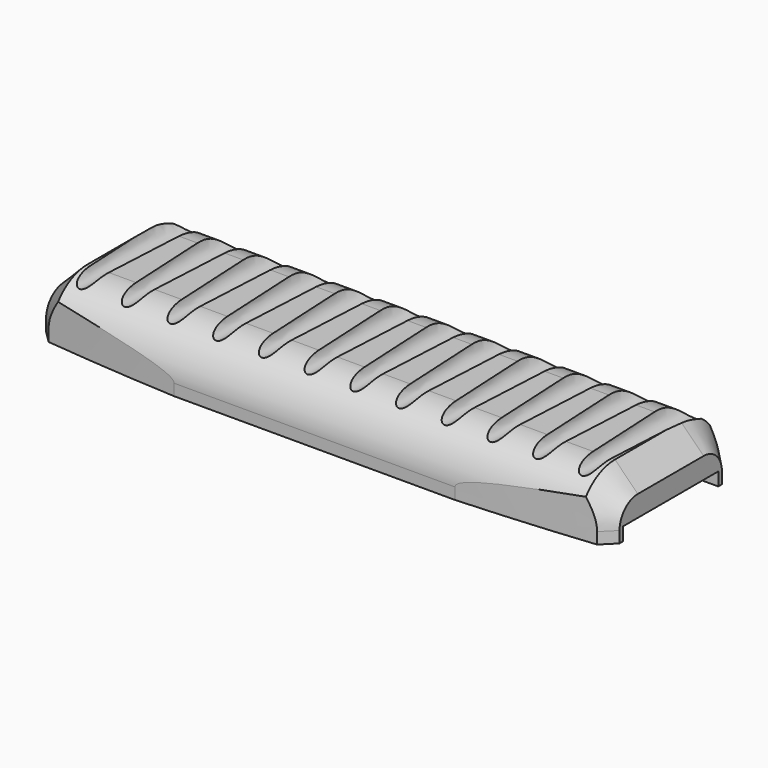
from build123d import *

# Parameters (mm, degrees)
F0_W         = 125.463343301
F0_H         = 38
F1_DEPTH     = 12.5
F2_W         = 26
F2_H         = 2.9014106728
F3_DEPTH     = 98.4
F4_R         = 10
F5_R         = 1.5
F6_DEPTH     = 42.5
F6_TAPER     = -3
F7_T1_DEPTH  = 15.3584149398
F7_T3_DEPTH  = 18
F7_T6_ANGLE  = 90
F7_T8_ANGLE  = 90
F7_T10_ANGLE = 90
F7_T12_ANGLE = 90
F9_DEPTH     = 25


# Not quite as in the source:
# - a fillet or chamfer that OpenCascade refuses, or shapes differently, is made with other operations: its cross-section is extruded or revolved along the edge and cut away or added


with BuildPart() as f1:
    # F0 (on Top) → F1 (new body)
    with BuildSketch(Plane.XY):
        with Locations((20.3044549349, 19)):
            Rectangle(F0_W, F0_H)
    extrude(amount=F1_DEPTH)

    # F2 (on Right) → F3 (cut, symmetric)
    with BuildSketch(Plane.YZ):
        with Locations((19, 1.4507053364)):
            Rectangle(F2_W, F2_H)
    extrude(amount=F3_DEPTH, both=True, mode=Mode.SUBTRACT)

    # F4
    f4_edges = [f1.edges().sort_by_distance(p)[0] for p in [
        (20.304455, 38, 12.5),
        (20.304455, 0, 12.5),
    ]]
    fillet(f4_edges, radius=F4_R)

    # F5 (on Front) → F6 (cut)
    with BuildSketch(Plane.XZ):
        with Locations((-34.7272167156, 12.6250582502)):
            Circle(F5_R)
        with Locations((-24.7272167156, 12.5)):
            Circle(F5_R)
        with Locations((-14.7272167156, 12.5)):
            Circle(F5_R)
        with Locations((-4.7272167156, 12.5)):
            Circle(F5_R)
        with Locations((5.2727832844, 12.5)):
            Circle(F5_R)
        with Locations((15.2727832844, 12.5)):
            Circle(F5_R)
        with Locations((25.2727832844, 12.5)):
            Circle(F5_R)
        with Locations((35.2727832844, 12.5)):
            Circle(F5_R)
        with Locations((45.2727832844, 12.5)):
            Circle(F5_R)
        with Locations((55.2727832844, 12.5)):
            Circle(F5_R)
        with Locations((65.2727832844, 12.5)):
            Circle(F5_R)
        with Locations((75.2727832844, 12.5)):
            Circle(F5_R)
    extrude(amount=-F6_DEPTH, taper=F6_TAPER, mode=Mode.SUBTRACT)

    # F7: chamfer of 5 on 2 edges, made by hand

    # F7_s2 → F7_t1 (cut)
    with BuildSketch(Plane.XY.offset(-12.8584149398)):
        Polygon((-37.4272167156, 38), (-42.4272167156, 33), (-42.4272167156, 38), align=None)
        Polygon((78.0361265854, 38), (83.0361265854, 33), (83.0361265854, 38), align=None)
        Polygon((78.0361265854, 0), (83.0361265854, 5), (83.0361265854, 0), align=None)
        Polygon((-42.4272167156, 5), (-37.4272167156, 0), (-42.4272167156, 0), align=None)
    extrude(amount=F7_T1_DEPTH, mode=Mode.SUBTRACT)

    # F7_s4 → F7_t3 (cut)
    with BuildSketch(Plane.XZ.offset(-28)):
        Polygon((78.0361265854, 12.5), (83.0361265854, 7.5), (83.0361265854, 12.5), align=None)
        Polygon((-42.4272167156, 7.5), (-37.4272167156, 12.5), (-42.4272167156, 12.5), align=None)
    extrude(amount=F7_T3_DEPTH, mode=Mode.SUBTRACT)

    # F7_s5 → F7_t6 (revolve, cut)
    with BuildSketch(Plane.XY.offset(2.5)):
        Polygon((78.0361265854, 38), (83.0361265854, 33), (83.0361265854, 38), align=None)
    revolve(axis=Axis((83.0361265854, 28, 2.5), (1, 0, 0)), revolution_arc=F7_T6_ANGLE, mode=Mode.SUBTRACT)

    # F7_s7 → F7_t8 (revolve, cut)
    with BuildSketch(Plane.XZ.offset(-10)):
        Polygon((78.0361265854, 12.5), (83.0361265854, 7.5), (83.0361265854, 12.5), align=None)
    revolve(axis=Axis((83.0361265854, 10, 2.5), (1, 0, 0)), revolution_arc=F7_T8_ANGLE, mode=Mode.SUBTRACT)

    # F7_s9 → F7_t10 (revolve, cut)
    with BuildSketch(Plane.XY.offset(2.5)):
        Polygon((-42.4272167156, 33), (-37.4272167156, 38), (-42.4272167156, 38), align=None)
    revolve(axis=Axis((-42.4272167156, 28, 2.5), (1, 0, 0)), revolution_arc=F7_T10_ANGLE, mode=Mode.SUBTRACT)

    # F7_s11 → F7_t12 (revolve, cut)
    with BuildSketch(Plane.XZ.offset(-10)):
        Polygon((-42.4272167156, 7.5), (-37.4272167156, 12.5), (-42.4272167156, 12.5), align=None)
    revolve(axis=Axis((-42.4272167156, 10, 2.5), (1, 0, 0)), revolution_arc=F7_T12_ANGLE, mode=Mode.SUBTRACT)

    # F6_face (on face) + F8 (on Top) → F9 (cut)
    with BuildSketch(Plane(origin=(-19.7272167156, 18.4349570526, 12.5), x_dir=(1, 0, 0), z_dir=(0, 0, 1))):
        with BuildLine():
            Line((2.0325821801, 9.5650429474), (-2.0325821801, 9.5650429474))
            add(Edge.make_bspline(
                [(-2.9759222072, -8.4349570525), (-2.0325821801, 9.5650429475)],
                knots=[0, 0, 1, 1], degree=1))
            Line((-2.9759222072, -8.4349570526), (2.9759222072, -8.4349570526))
            Line((2.9759222072, -8.4349570526), (2.0325821801, 9.5650429474))
        make_face()
    with BuildSketch(Plane.XY):
        with BuildLine():
            Line((95.2727832844, 48), (-54.7272167156, 48))
            Line((-54.7272167156, 48), (-54.7272167156, 33.9810573746))
            ThreePointArc((-54.7272167156, 33.9810573746), (20.2725203798, 38.8069620788), (95.2727832844, 33.9892359715))
            Line((95.2727832844, 33.9892359715), (95.2727832844, 48))
        make_face()
        with BuildLine():
            ThreePointArc((95.2727832844, 4.0107601545), (20.2725203794, -0.806969631), (-54.7272167156, 4.0189387577))
            Line((-54.7272167156, 4.0189387577), (-54.7272167156, -10))
            Line((-54.7272167156, -10), (95.2727832844, -10))
            Line((95.2727832844, -10), (95.2727832844, 4.0107601545))
        make_face()
    extrude(amount=F9_DEPTH, mode=Mode.SUBTRACT)


solid = f1.part
